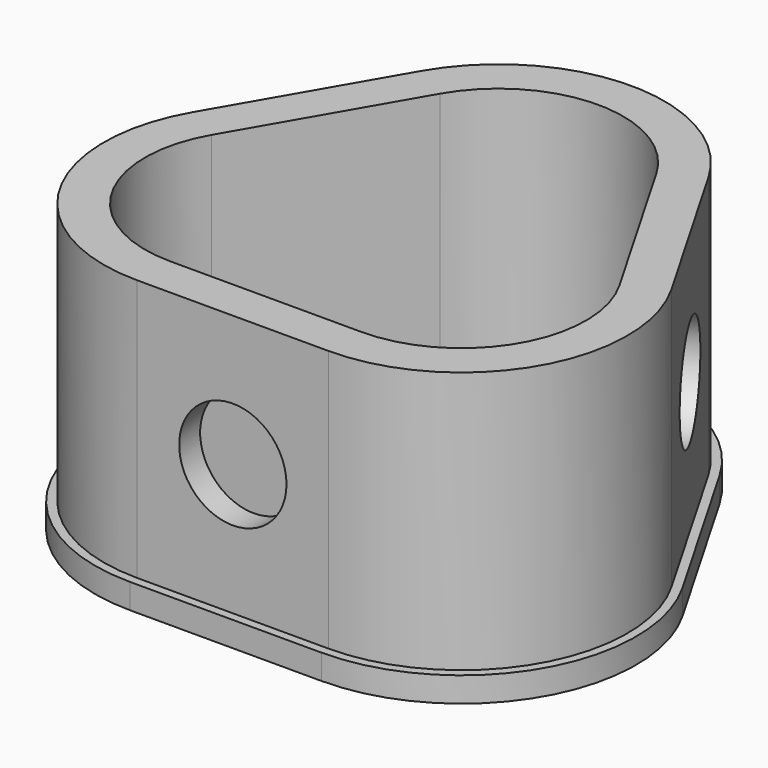
from build123d import *

# Parameters (mm, degrees)
F1_DEPTH        = 25
F3_START        = -0.65
F2_R            = 4.3
F3_DEPTH        = 2.15
F3_COPIES_COUNT = 3
F6_R            = 33.7024135389
F7_DEPTH        = 2
F9_DEPTH        = 21


# Not quite as in the source:
# - a pattern or mirror of a feature is missing from the dataset's text; its kind, count and spacing are read off the source's solid


with BuildPart() as f1:
    # F0 (on Top) → F1 (new body)
    with BuildSketch(Plane.XY):
        with BuildLine():
            ThreePointArc((7.6794919243, -4), (19.8038475773, 3), (19.8038475773, 17))
            Line((19.8038475773, 17), (12.124355653, 30.3012701892))
            ThreePointArc((12.124355653, 30.3012701892), (0, 37.3012701892), (-12.124355653, 30.3012701892))
            Line((-12.124355653, 30.3012701892), (-19.8038475773, 17))
            ThreePointArc((-19.8038475773, 17), (-19.8038475773, 3), (-7.6794919243, -4))
            Line((-7.6794919243, -4), (0, -4))
            Line((0, -4), (7.6794919243, -4))
        make_face()
        with BuildLine():
            Line((7.6794919243, 0), (0, 0))
            Line((0, 0), (-7.6794919243, 0))
            ThreePointArc((-7.6794919243, 0), (-16.3397459622, 5), (-16.3397459622, 15))
            Line((-16.3397459622, 15), (-8.6602540378, 28.3012701892))
            ThreePointArc((-8.6602540378, 28.3012701892), (0, 33.3012701892), (8.6602540378, 28.3012701892))
            Line((8.6602540378, 28.3012701892), (16.3397459622, 15))
            ThreePointArc((16.3397459622, 15), (16.3397459622, 5), (7.6794919243, 0))
        make_face(mode=Mode.SUBTRACT)
    extrude(amount=F1_DEPTH)

    # F2 (on face) → F3 (cut)
    with BuildSketch(Plane(origin=(-22.2141016151, 12.8253175473, 0), x_dir=(-0.5, -0.8660254038, 0), z_dir=(-0.8660254038, 0.5, 0)).offset(F3_START)):
        with Locations((-12.5, 12.5)):
            Circle(F2_R)
    f3 = extrude(amount=-F3_DEPTH, mode=Mode.SUBTRACT)

    # F3_copies: F3 ×3 about axis
    f3_copies_axis = Axis((0, 14.433757, 0), (0, 0, 1))
    for i in range(1, F3_COPIES_COUNT):
        add(f3.rotate(f3_copies_axis, i * 360 / F3_COPIES_COUNT), mode=Mode.SUBTRACT)

    # F6 (on face) → F7 (cut)
    with BuildSketch(Plane.XY.offset(25)):
        with Locations((0, 15.2027085423)):
            Circle(F6_R)
    extrude(amount=-F7_DEPTH, mode=Mode.SUBTRACT)

    # F8 (on face) → F9 (cut)
    with BuildSketch(Plane.XY.offset(23)):
        with BuildLine():
            Line((-12.124355653, 30.3012701892), (-19.8038475773, 17))
            ThreePointArc((-19.8038475773, 17), (-19.8038475773, 3), (-7.6794919243, -4))
            Line((-7.6794919243, -4), (7.6794919243, -4))
            ThreePointArc((7.6794919243, -4), (19.8038475773, 3), (19.8038475773, 17))
            Line((19.8038475773, 17), (12.124355653, 30.3012701892))
            ThreePointArc((12.124355653, 30.3012701892), (0, 37.3012701892), (-12.124355653, 30.3012701892))
        make_face()
        with BuildLine():
            ThreePointArc((-11.5181378703, 29.9512701892), (0, 36.6012701892), (11.5181378703, 29.9512701892))
            Line((11.5181378703, 29.9512701892), (19.1976297946, 16.65))
            ThreePointArc((19.1976297946, 16.65), (19.1976297946, 3.35), (7.6794919243, -3.3))
            Line((7.6794919243, -3.3), (-7.6794919243, -3.3))
            ThreePointArc((-7.6794919243, -3.3), (-19.1976297946, 3.35), (-19.1976297946, 16.65))
            Line((-19.1976297946, 16.65), (-11.5181378703, 29.9512701892))
        make_face(mode=Mode.SUBTRACT)
    extrude(amount=-F9_DEPTH, mode=Mode.SUBTRACT)


solid = f1.part
